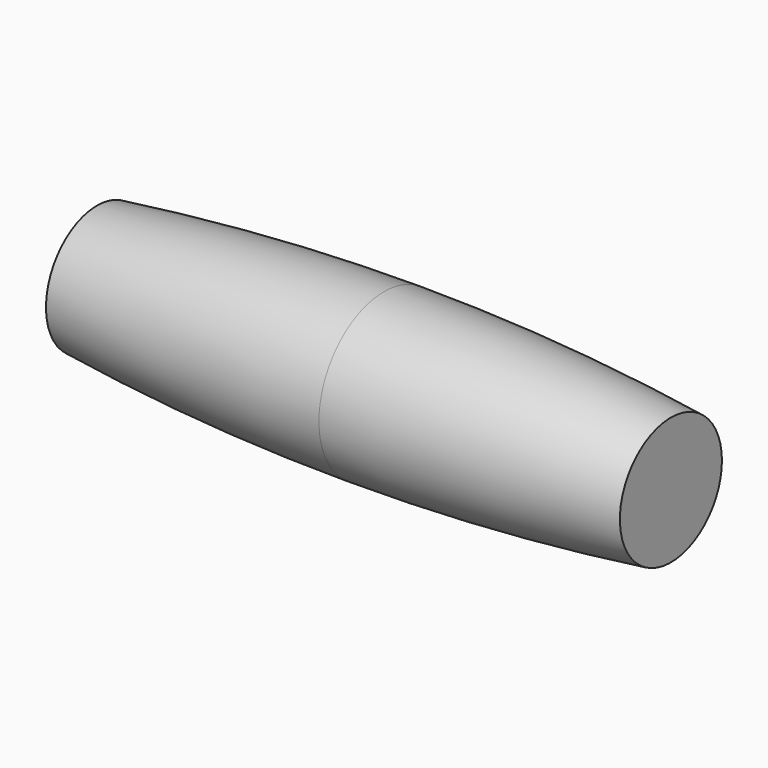
from build123d import *


with BuildPart() as f1:
    # F0 (on Top) → F1 (revolve)
    with BuildSketch(Plane.XY):
        with BuildLine():
            Line((45, 12.75), (45, 0))
            Line((45, 0), (90, 0))
            Line((90, 0), (90, 10))
            ThreePointArc((90, 10), (67.541974736, 12.0618593169), (45, 12.75))
        make_face()
        with BuildLine():
            Line((0, 10), (0, 0))
            Line((0, 0), (45, 0))
            Line((45, 0), (45, 12.75))
            ThreePointArc((45, 12.75), (22.458025264, 12.0618593169), (0, 10))
        make_face()
    revolve(axis=Axis((45, 0, 0), (1, 0, 0)))


solid = f1.part
